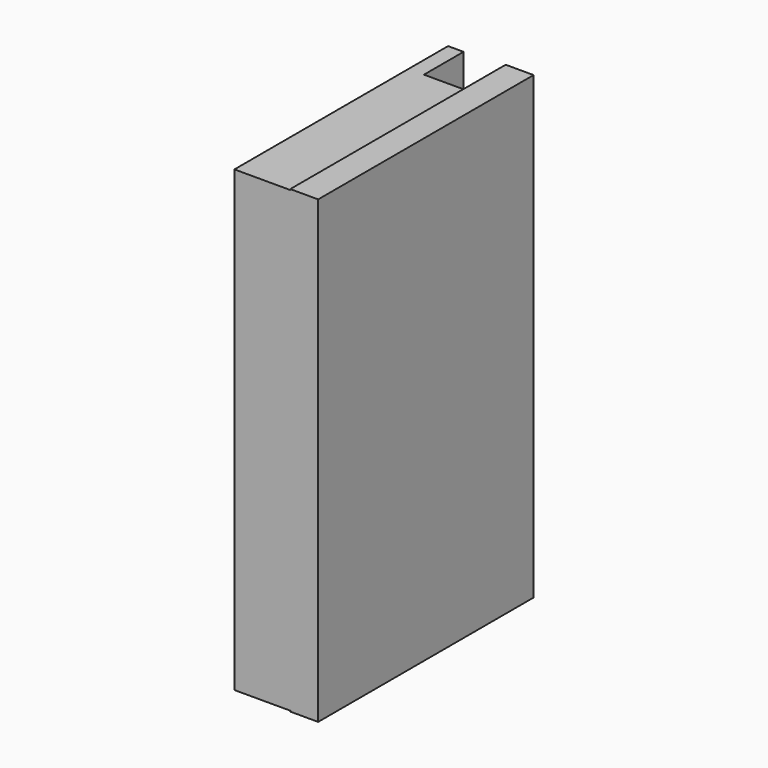
from build123d import *

# Parameters (mm, degrees)
F0_W     = 43.7379740179
F0_H     = 75.0739984214
F1_DEPTH = 2.54
F2_W     = 35.6321558356
F2_H     = 75.0739984214
F3_DEPTH = 6.604
F4_W     = 44.1027786583
F4_H     = 75.3439329565
F5_DEPTH = 4.572


# Not quite as in the source:
# - the program builds the solid bodies; features that only make, move or delete a surface that nothing else refers to are left out


with BuildPart() as f1:
    # F0 (on Right) → F1 (new body)
    with BuildSketch(Plane.YZ):
        with Locations((-2.128392458, 14.8043204099)):
            Rectangle(F0_W, F0_H)
    extrude(amount=F1_DEPTH)

    # F2 (on face) → F3 (join)
    with BuildSketch(Plane.YZ.offset(2.54)):
        with Locations((-6.1813015491, 14.8043204099)):
            Rectangle(F2_W, F2_H)
    extrude(amount=F3_DEPTH)

    # F4 (on face) → F5 (join)
    with BuildSketch(Plane.YZ.offset(9.144)):
        with Locations((-1.9459901378, 14.8043166846)):
            Rectangle(F4_W, F4_H)
    extrude(amount=F5_DEPTH)


solid = f1.part
